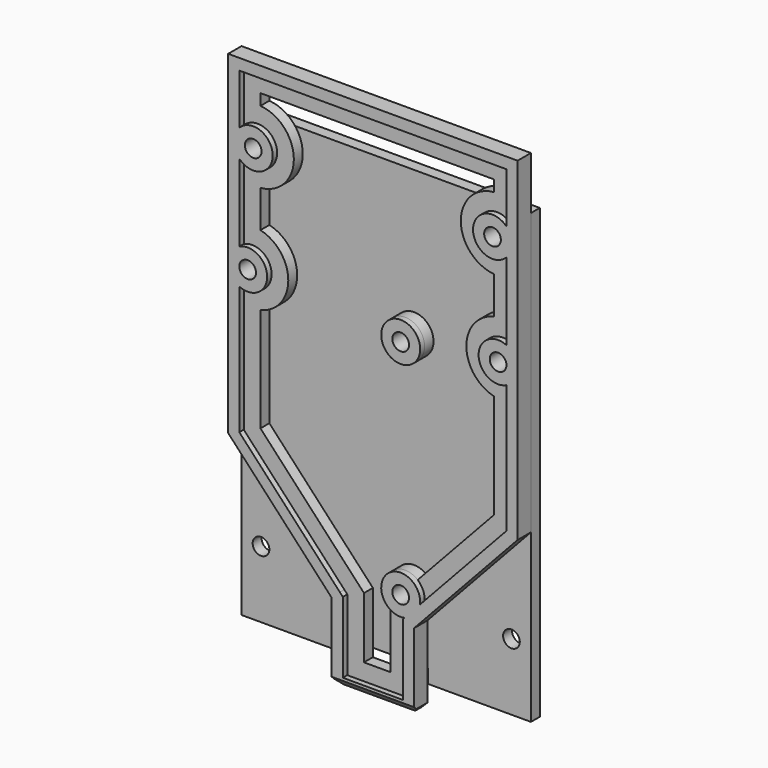
from build123d import *

# Parameters (mm, degrees)
F0_R        = 1.5
F1_DEPTH    = 2
F2_W        = 52
F2_H        = 9.5
F2_R        = 1.5
F2_W_2      = 14.8
F2_H_2      = 2.5
F3_DEPTH    = 3
F4_T        = 2
F4_T3_DEPTH = 7
F5_SIZE     = 1.5
F6_SIZE     = 1
F7_R        = 3.5
F8_DEPTH    = 25


# Not quite as in the source:
# - a shell that OpenCascade refuses in one call is made with other operations: the cavity is built on its own and cut out


with BuildPart() as f1:
    # F0 (on Front) → F1 (new body)
    with BuildSketch(Plane.XZ):
        Polygon((26, -40.25), (26, 40.25), (-26, 40.25), (-26, -40.25), (-7.5, -40.25), (-7.5, -37.75), (7.5, -37.75), (7.5, -40.25), align=None)
        with Locations((-22.5, -28.25)):
            Circle(F0_R, mode=Mode.SUBTRACT)
        with Locations((5, -25.75)):
            Circle(F0_R, mode=Mode.SUBTRACT)
        with Locations((22.5, -28.25)):
            Circle(F0_R, mode=Mode.SUBTRACT)
        with Locations((-22.5, 16.75)):
            Circle(F0_R, mode=Mode.SUBTRACT)
        with Locations((-21.5, 36.25)):
            Circle(F0_R, mode=Mode.SUBTRACT)
        with Locations((5, 14.25)):
            Circle(F0_R, mode=Mode.SUBTRACT)
        with Locations((22.5, 16.75)):
            Circle(F0_R, mode=Mode.SUBTRACT)
        with Locations((21.5, 36.25)):
            Circle(F0_R, mode=Mode.SUBTRACT)
    extrude(amount=-F1_DEPTH)


with BuildPart() as f3:
    # F2 (on face) → F3 (new body)
    with BuildSketch(Plane.XZ):
        Polygon((7.4, -40.25), (-7.4, -40.25), (-7.4, -44.25), (0, -44.25), (7.4, -44.25), align=None)
        with Locations((0, 45)):
            Rectangle(F2_W, F2_H)
        Polygon((-26, 40.25), (-26, -10.25), (-7.4, -30.25), (-7.4, -37.75), (7.4, -37.75), (7.4, -30.25), (26, -10.25), (26, 40.25), align=None)
        with Locations((5, -25.75)):
            Circle(F2_R, mode=Mode.SUBTRACT)
        with Locations((-22.5, 16.75)):
            Circle(F2_R, mode=Mode.SUBTRACT)
        with Locations((-21.5, 36.25)):
            Circle(F2_R, mode=Mode.SUBTRACT)
        with Locations((5, 14.25)):
            Circle(F2_R, mode=Mode.SUBTRACT)
        with Locations((22.5, 16.75)):
            Circle(F2_R, mode=Mode.SUBTRACT)
        with Locations((21.5, 36.25)):
            Circle(F2_R, mode=Mode.SUBTRACT)
        with Locations((0, -39)):
            Rectangle(F2_W_2, F2_H_2)
    extrude(amount=F3_DEPTH)

    # F4: shell of thickness 2, made by hand


with BuildPart() as f4_core1:
    # F4_t2: copy of F3
    add(f3.part)

    # the walls: a layer under each face that stays
    f4_faces = [f4_core1.faces().sort_by_distance(p)[0] for p in [
        (0, -1.5, -44.25),
        (7.4, -1.5, -37.25),
        (16.7, -1.5, -20.25),
        (26, -1.5, 19.75),
        (0, -1.5, 49.75),
        (-26, -1.5, 19.75),
        (-16.7, -1.5, -20.25),
        (-7.4, -1.5, -37.25),
        (21, -1.5, 16.75),
        (20, -1.5, 36.25),
        (3.5, -1.5, -25.75),
        (-24, -1.5, 16.75),
        (-23, -1.5, 36.25),
        (3.5, -1.5, 14.25),
        (0, 0, 2.75),
    ]]
    thicken(f4_faces, amount=-F4_T, mode=Mode.SUBTRACT)

    # F4_s4 → F4_t3 (cut)
    with BuildSketch(Plane.XZ.offset(-2)):
        Polygon((7.4346454332, -30.2636202528), (5.4, -30.25), (5.4, -29.4637345908), (5.9354566837, -28.8879747158), align=None)
        Polygon((-7.4346454332, -30.2636202528), (-5.9354566837, -28.8879747158), (-5.4, -29.4637345908), (-5.4, -30.25), align=None)
    extrude(amount=F4_T3_DEPTH, mode=Mode.SUBTRACT)


with BuildPart() as f3_1:
    add(f3.part)

    # what is left inside the walls is the cavity
    f4_cavity = [f4_core1.part.solids().sort_by_distance(p)[0] for p in [
        (0, -2.98, -12.25),
    ]]
    add(f4_cavity, mode=Mode.SUBTRACT)

    # F5
    f5_edges = [f3_1.edges().sort_by_distance(p)[0] for p in [
        (0, -3, -44.25),
    ]]
    chamfer(f5_edges, length=F5_SIZE)

    # F6
    f6_edges = [f3_1.edges().sort_by_distance(p)[0] for p in [
        (-7.4, -0.75, -44.25),
        (7.4, -0.75, -44.25),
    ]]
    chamfer(f6_edges, length=F6_SIZE)

    # F7 (on face) → F8 (cut)
    with BuildSketch(Plane.XZ.offset(2)):
        with BuildLine():
            Line((21, -8.284336477), (21, 10.4254446797))
            ThreePointArc((21, 10.4254446797), (16, 16.75), (21, 23.0745553203))
            Line((21, 23.0745553203), (21, 29.7692593016))
            ThreePointArc((21, 29.7692593016), (15, 36.25), (21, 42.7307406984))
            Line((21, 42.7307406984), (21, 44.75))
            Line((21, 44.75), (-21, 44.75))
            Line((-21, 44.75), (-21, 42.7307406984))
            ThreePointArc((-21, 42.7307406984), (-15, 36.25), (-21, 29.7692593016))
            Line((-21, 29.7692593016), (-21, 23.0745553203))
            ThreePointArc((-21, 23.0745553203), (-16, 16.75), (-21, 10.4254446797))
            Line((-21, 10.4254446797), (-21, -8.284336477))
            Line((-21, -8.284336477), (-2.4, -28.284336477))
            Line((-2.4, -28.284336477), (-2.4, -39.25))
            Line((-2.4, -39.25), (2.4, -39.25))
            Line((2.4, -39.25), (2.4, -28.284336477))
            Line((2.4, -28.284336477), (2.489202038, -28.1884203071))
            ThreePointArc((2.489202038, -28.1884203071), (2.4370491965, -23.3664557527), (7.2501222406, -23.069151272))
            Line((7.2501222406, -23.069151272), (21, -8.284336477))
        make_face()
        with Locations((5, 14.25)):
            Circle(F7_R, mode=Mode.SUBTRACT)
    extrude(amount=-F8_DEPTH, mode=Mode.SUBTRACT)


solid = Compound([f1.part, f3_1.part])
